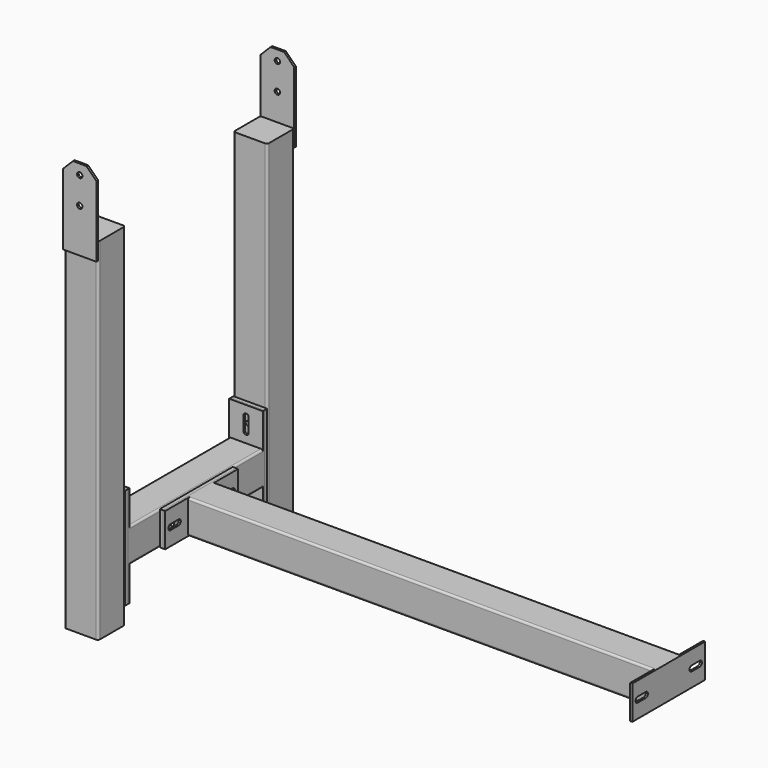
from build123d import *

# Parameters (mm, degrees)
F1_DEPTH  = 520
F2_W      = 50
F2_H      = 150
F2_R      = 3
F3_DEPTH  = 5
F5_DEPTH  = 1.5
F6_W      = 50
F6_H      = 120
F6_R      = 4
F7_DEPTH  = 3
F8_SIZE   = 15
F11_W     = 50
F11_H     = 150
F12_DEPTH = 3
F15_DEPTH = 247
F17_W     = 135
F17_H     = 50
F17_R     = 3
F18_DEPTH = 5
F19_W     = 135
F19_H     = 50
F19_R     = 4
F20_DEPTH = 3
F23_DEPTH = 689
F25_DEPTH = 3.001


# Not quite as in the source:
# - a pattern or mirror of a feature is missing from the dataset's text; its kind, count and spacing are read off the source's solid


with BuildPart() as f1:
    # F0 (on Top) → F1 (new body)
    with BuildSketch(Plane.XY):
        with BuildLine():
            Line((-22, -25), (22, -25))
            ThreePointArc((22, -25), (24.1213203436, -24.1213203436), (25, -22))
            Line((25, -22), (25, 22))
            ThreePointArc((25, 22), (24.1213203436, 24.1213203436), (22, 25))
            Line((22, 25), (-22, 25))
            ThreePointArc((-22, 25), (-24.1213203436, 24.1213203436), (-25, 22))
            Line((-25, 22), (-25, -22))
            ThreePointArc((-25, -22), (-24.1213203436, -24.1213203436), (-22, -25))
        make_face()
        with BuildLine():
            ThreePointArc((22, 23.5), (23.0606601718, 23.0606601718), (23.5, 22))
            Line((23.5, 22), (23.5, -22))
            ThreePointArc((23.5, -22), (23.0606601718, -23.0606601718), (22, -23.5))
            Line((22, -23.5), (-22, -23.5))
            ThreePointArc((-22, -23.5), (-23.0606601718, -23.0606601718), (-23.5, -22))
            Line((-23.5, -22), (-23.5, 22))
            ThreePointArc((-23.5, 22), (-23.0606601718, 23.0606601718), (-22, 23.5))
            Line((-22, 23.5), (22, 23.5))
        make_face(mode=Mode.SUBTRACT)
    extrude(amount=F1_DEPTH)

    # F2 (on face) → F3 (join)
    with BuildSketch(Plane(origin=(0, 25, 0), x_dir=(-1, 0, 0), z_dir=(0, 1, 0))):
        with Locations((0, 100)):
            Rectangle(F2_W, F2_H)
        with Locations((0, 50)):
            Circle(F2_R, mode=Mode.SUBTRACT)
        with Locations((0, 150)):
            Circle(F2_R, mode=Mode.SUBTRACT)
    extrude(amount=F3_DEPTH)

    # F4 (on face) → F5 (join)
    with BuildSketch(Plane.XY.offset(520)):
        with BuildLine():
            ThreePointArc((23.5, 22), (23.0606601718, 23.0606601718), (22, 23.5))
            Line((22, 23.5), (-22, 23.5))
            ThreePointArc((-22, 23.5), (-23.0606601718, 23.0606601718), (-23.5, 22))
            Line((-23.5, 22), (-23.5, -22))
            ThreePointArc((-23.5, -22), (-23.0606601718, -23.0606601718), (-22, -23.5))
            Line((-22, -23.5), (22, -23.5))
            ThreePointArc((22, -23.5), (23.0606601718, -23.0606601718), (23.5, -22))
            Line((23.5, -22), (23.5, 22))
        make_face()
    extrude(amount=-F5_DEPTH)

    # F6 (on face) → F7 (join)
    with BuildSketch(Plane.XZ.offset(25)):
        with Locations((0, 555)):
            Rectangle(F6_W, F6_H)
        with Locations((0, 560)):
            Circle(F6_R, mode=Mode.SUBTRACT)
        with Locations((0, 600)):
            Circle(F6_R, mode=Mode.SUBTRACT)
    extrude(amount=F7_DEPTH)

    # F8
    f8_edges = [f1.edges().sort_by_distance(p)[0] for p in [
        (25, -26.5, 615),
        (-25, -26.5, 615),
    ]]
    chamfer(f8_edges, length=F8_SIZE)


with BuildPart() as f10_1:
    # F10: instance of F1
    add(f1.part.mirror(Plane(origin=(0, 156.5, 563.1674453561), x_dir=(1, 0, 0), z_dir=(0, 1, 0))))


with BuildPart() as f12:
    # F11 (on face) → F12 (new body)
    with BuildSketch(Plane(origin=(0, 30, 0), x_dir=(-1, 0, 0), z_dir=(0, 1, 0))):
        with Locations((0, 100)):
            Rectangle(F11_W, F11_H)
        with BuildLine():
            Line((-4, 40), (-4, 60))
            ThreePointArc((-4, 60), (0, 64), (4, 60))
            Line((4, 60), (4, 40))
            ThreePointArc((4, 40), (0, 36), (-4, 40))
        make_face(mode=Mode.SUBTRACT)
        with BuildLine():
            Line((4, 160), (4, 140))
            ThreePointArc((4, 140), (0, 136), (-4, 140))
            Line((-4, 140), (-4, 160))
            ThreePointArc((-4, 160), (0, 164), (4, 160))
        make_face(mode=Mode.SUBTRACT)
    extrude(amount=F12_DEPTH)


with BuildPart() as f13_1:
    # F13: instance of F12
    add(f12.part.mirror(Plane(origin=(0, 156.5, 563.1674453561), x_dir=(1, 0, 0), z_dir=(0, 1, 0))))


with BuildPart() as f12_1:
    add(f12.part)

    add(f13_1.part)  # F15 merges F13_1
    # F14 (on face) → F15 (join, through all)
    with BuildSketch(Plane(origin=(0, 33, 0), x_dir=(-1, 0, 0), z_dir=(0, 1, 0))):
        with BuildLine():
            Line((-22, 75), (22, 75))
            ThreePointArc((22, 75), (24.1213203436, 75.8786796564), (25, 78))
            Line((25, 78), (25, 122))
            ThreePointArc((25, 122), (24.1213203436, 124.1213203436), (22, 125))
            Line((22, 125), (-22, 125))
            ThreePointArc((-22, 125), (-24.1213203436, 124.1213203436), (-25, 122))
            Line((-25, 122), (-25, 78))
            ThreePointArc((-25, 78), (-24.1213203436, 75.8786796564), (-22, 75))
        make_face()
        with BuildLine():
            ThreePointArc((22, 123.5), (23.0606601718, 123.0606601718), (23.5, 122))
            Line((23.5, 122), (23.5, 78))
            ThreePointArc((23.5, 78), (23.0606601718, 76.9393398282), (22, 76.5))
            Line((22, 76.5), (-22, 76.5))
            ThreePointArc((-22, 76.5), (-23.0606601718, 76.9393398282), (-23.5, 78))
            Line((-23.5, 78), (-23.5, 122))
            ThreePointArc((-23.5, 122), (-23.0606601718, 123.0606601718), (-22, 123.5))
            Line((-22, 123.5), (22, 123.5))
        make_face(mode=Mode.SUBTRACT)
    extrude(amount=F15_DEPTH)

    # F17 (on face) → F18 (join)
    with BuildSketch(Plane.YZ.offset(25)):
        with Locations((156.5, 100)):
            Rectangle(F17_W, F17_H)
        with Locations((106.5, 100)):
            Circle(F17_R, mode=Mode.SUBTRACT)
        with Locations((206.5, 100)):
            Circle(F17_R, mode=Mode.SUBTRACT)
    extrude(amount=F18_DEPTH)


with BuildPart() as f20:
    # F19 (on face) → F20 (new body)
    with BuildSketch(Plane.YZ.offset(30)):
        with Locations((156.5, 100)):
            Rectangle(F19_W, F19_H)
        with Locations((106.5, 100)):
            Circle(F19_R, mode=Mode.SUBTRACT)
        with Locations((206.5, 100)):
            Circle(F19_R, mode=Mode.SUBTRACT)
    extrude(amount=F20_DEPTH)


with BuildPart() as f21_1:
    # F21: instance of F20
    add(f20.part.mirror(Plane(origin=(377.5, 0, 260), x_dir=(0, 1, 0), z_dir=(1, 0, 0))))


with BuildPart() as f20_1:
    add(f20.part)

    add(f21_1.part)  # F23 merges F21_1
    # F22 (on face) → F23 (join, through all)
    with BuildSketch(Plane.YZ.offset(33)):
        with BuildLine():
            Line((134.5, 75), (178.5, 75))
            ThreePointArc((178.5, 75), (180.6213203436, 75.8786796564), (181.5, 78))
            Line((181.5, 78), (181.5, 122))
            ThreePointArc((181.5, 122), (180.6213203436, 124.1213203436), (178.5, 125))
            Line((178.5, 125), (134.5, 125))
            ThreePointArc((134.5, 125), (132.3786796564, 124.1213203436), (131.5, 122))
            Line((131.5, 122), (131.5, 78))
            ThreePointArc((131.5, 78), (132.3786796564, 75.8786796564), (134.5, 75))
        make_face()
        with BuildLine():
            ThreePointArc((178.5, 123.5), (179.5606601718, 123.0606601718), (180, 122))
            Line((180, 122), (180, 78))
            ThreePointArc((180, 78), (179.5606601718, 76.9393398282), (178.5, 76.5))
            Line((178.5, 76.5), (134.5, 76.5))
            ThreePointArc((134.5, 76.5), (133.4393398282, 76.9393398282), (133, 78))
            Line((133, 78), (133, 122))
            ThreePointArc((133, 122), (133.4393398282, 123.0606601718), (134.5, 123.5))
            Line((134.5, 123.5), (178.5, 123.5))
        make_face(mode=Mode.SUBTRACT)
    extrude(amount=F23_DEPTH)

    # F24 (on face) → F25 (cut, through all)
    with BuildSketch(Plane.YZ.offset(725)):
        with BuildLine():
            Line((99, 96), (114, 96))
            ThreePointArc((114, 96), (118, 100), (114, 104))
            Line((114, 104), (99, 104))
            ThreePointArc((99, 104), (95, 100), (99, 96))
        make_face()
        with BuildLine():
            ThreePointArc((199, 104), (195, 100), (199, 96))
            Line((199, 96), (214, 96))
            ThreePointArc((214, 96), (218, 100), (214, 104))
            Line((214, 104), (199, 104))
        make_face()
    f25 = extrude(amount=-F25_DEPTH, mode=Mode.SUBTRACT)

    # F25_copies: F25 across plane
    add(f25.mirror(Plane(origin=(377.5, 0, 0), x_dir=(0, 0, -1), z_dir=(-1, 0, 0))), mode=Mode.SUBTRACT)


solid = Compound([f1.part, f10_1.part, f12_1.part, f20_1.part])
